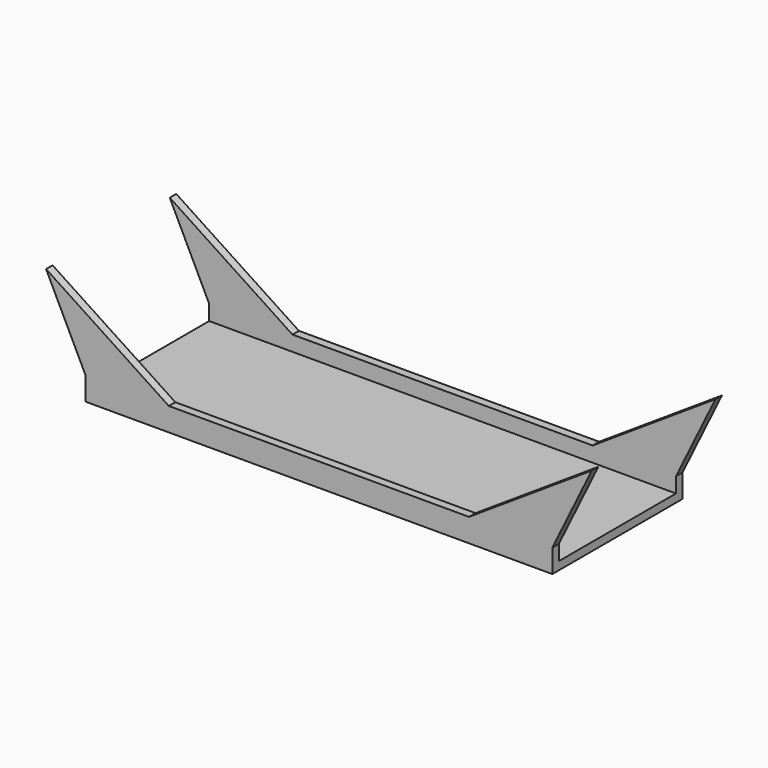
from build123d import *

# Parameters (mm, degrees)
F1_DEPTH = 50.8
F2_DEPTH = 50.8
F4_T     = -2.54


with BuildPart() as f1:
    # F0 (on Front) → F1 (new body)
    with BuildSketch(Plane.XZ):
        Polygon((-85.1854681969, 35.1092815399), (-72.8762447834, 9.9313110113), (-46.8590036035, 9.9313110113), align=None)
    extrude(amount=F1_DEPTH)

    # F0 (on Front) → F2 (join)
    with BuildSketch(Plane.XZ):
        Polygon((-46.8590036035, 9.9313110113), (-72.8762447834, 9.9313110113), (-72.8762447834, 2.6576747186), (48.8172881305, 2.6576747186), (48.8172881305, 9.9313110113), align=None)
    extrude(amount=F2_DEPTH)

    # F3: F1 across plane


with BuildPart() as f1_1:
    add(f1.part)
    add(f1.part.mirror(Plane.YZ))

    # F4
    f4_openings = [f1_1.faces().sort_by_distance(p)[0] for p in [
        (-66.022236, -25.4, 22.520296),
        (79.030856, -25.4, 22.520296),
        (66.022236, -25.4, 22.520296),
        (-79.030856, -25.4, 22.520296),
        (0, -25.4, 9.931311),
        (72.876245, -25.4, 6.294493),
        (-72.876245, -25.4, 6.294493),
    ]]
    offset(amount=F4_T, openings=f4_openings)


solid = f1_1.part
